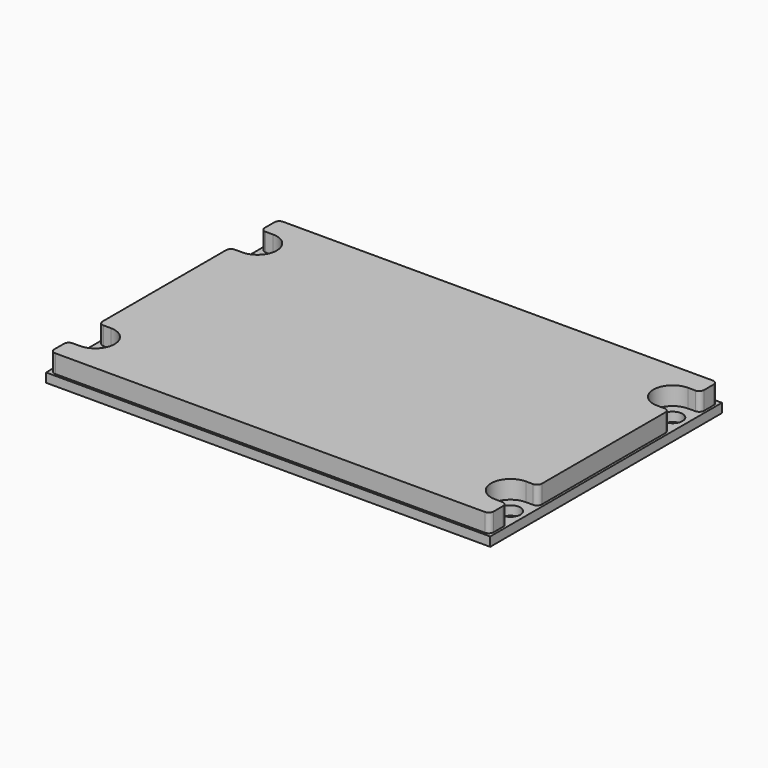
from build123d import *

# Parameters (mm, degrees)
F0_R     = 3.24
F1_DEPTH = 3
F2_DEPTH = 6
F3_R     = 1.588


# Not quite as in the source:
# - a feature names something its author has since deleted; it is built from what else it names


with BuildPart() as f1:
    # F0 (on Top) → F1 (new body)
    with BuildSketch(Plane.XY):
        Polygon((0, 57.15), (-73.025, 57.15), (-73.025, 9.525), (-73.025, -38.1), (73.025, -38.1), (73.025, 57.15), align=None)
        with Locations((-68.262, -23.812)):
            Circle(F0_R, mode=Mode.SUBTRACT)
        with Locations((68.262, -23.812)):
            Circle(F0_R, mode=Mode.SUBTRACT)
        with Locations((-68.262, 42.862)):
            Circle(F0_R, mode=Mode.SUBTRACT)
        with BuildLine():
            Line((-72.225, -17.461), (-72.225, 9.525))
            Line((-72.225, 9.525), (-72.225, 36.511))
            Line((-72.225, 36.511), (-68.262, 36.511))
            ThreePointArc((-68.262, 36.511), (-61.911, 42.862), (-68.262, 49.213))
            Line((-68.262, 49.213), (-72.225, 49.213))
            Line((-72.225, 49.213), (-72.225, 56.35))
            Line((-72.225, 56.35), (72.225, 56.35))
            Line((72.225, 56.35), (72.225, 49.213))
            Line((72.225, 49.213), (68.262, 49.213))
            ThreePointArc((68.262, 49.213), (61.911, 42.862), (68.262, 36.511))
            Line((68.262, 36.511), (72.225, 36.511))
            Line((72.225, 36.511), (72.225, -17.461))
            Line((72.225, -17.461), (68.262, -17.461))
            ThreePointArc((68.262, -17.461), (61.911, -23.812), (68.262, -30.163))
            Line((68.262, -30.163), (72.225, -30.163))
            Line((72.225, -30.163), (72.225, -37.3))
            Line((72.225, -37.3), (-72.225, -37.3))
            Line((-72.225, -37.3), (-72.225, -30.163))
            Line((-72.225, -30.163), (-68.262, -30.163))
            ThreePointArc((-68.262, -30.163), (-61.911, -23.812), (-68.262, -17.461))
            Line((-68.262, -17.461), (-72.225, -17.461))
        make_face(mode=Mode.SUBTRACT)
        with Locations((68.262, 42.862)):
            Circle(F0_R, mode=Mode.SUBTRACT)
        with BuildLine():
            Line((-72.225, 36.511), (-72.225, 9.525))
            Line((-72.225, 9.525), (-72.225, -17.461))
            Line((-72.225, -17.461), (-68.262, -17.461))
            ThreePointArc((-68.262, -17.461), (-61.911, -23.812), (-68.262, -30.163))
            Line((-68.262, -30.163), (-72.225, -30.163))
            Line((-72.225, -30.163), (-72.225, -37.3))
            Line((-72.225, -37.3), (72.225, -37.3))
            Line((72.225, -37.3), (72.225, -30.163))
            Line((72.225, -30.163), (68.262, -30.163))
            ThreePointArc((68.262, -30.163), (61.911, -23.812), (68.262, -17.461))
            Line((68.262, -17.461), (72.225, -17.461))
            Line((72.225, -17.461), (72.225, 36.511))
            Line((72.225, 36.511), (68.262, 36.511))
            ThreePointArc((68.262, 36.511), (61.911, 42.862), (68.262, 49.213))
            Line((68.262, 49.213), (72.225, 49.213))
            Line((72.225, 49.213), (72.225, 56.35))
            Line((72.225, 56.35), (-72.225, 56.35))
            Line((-72.225, 56.35), (-72.225, 49.213))
            Line((-72.225, 49.213), (-68.262, 49.213))
            ThreePointArc((-68.262, 49.213), (-61.911, 42.862), (-68.262, 36.511))
            Line((-68.262, 36.511), (-72.225, 36.511))
        make_face()
    extrude(amount=-F1_DEPTH)


with BuildPart() as f2:
    # F0 (on Top) → F2 (new body)
    with BuildSketch(Plane.XY):
        with BuildLine():
            Line((-72.225, 36.511), (-72.225, 9.525))
            Line((-72.225, 9.525), (-72.225, -17.461))
            Line((-72.225, -17.461), (-68.262, -17.461))
            ThreePointArc((-68.262, -17.461), (-61.911, -23.812), (-68.262, -30.163))
            Line((-68.262, -30.163), (-72.225, -30.163))
            Line((-72.225, -30.163), (-72.225, -37.3))
            Line((-72.225, -37.3), (72.225, -37.3))
            Line((72.225, -37.3), (72.225, -30.163))
            Line((72.225, -30.163), (68.262, -30.163))
            ThreePointArc((68.262, -30.163), (61.911, -23.812), (68.262, -17.461))
            Line((68.262, -17.461), (72.225, -17.461))
            Line((72.225, -17.461), (72.225, 36.511))
            Line((72.225, 36.511), (68.262, 36.511))
            ThreePointArc((68.262, 36.511), (61.911, 42.862), (68.262, 49.213))
            Line((68.262, 49.213), (72.225, 49.213))
            Line((72.225, 49.213), (72.225, 56.35))
            Line((72.225, 56.35), (-72.225, 56.35))
            Line((-72.225, 56.35), (-72.225, 49.213))
            Line((-72.225, 49.213), (-68.262, 49.213))
            ThreePointArc((-68.262, 49.213), (-61.911, 42.862), (-68.262, 36.511))
            Line((-68.262, 36.511), (-72.225, 36.511))
        make_face()
    extrude(amount=F2_DEPTH)

    # F3
    f3_edges = [f2.edges().sort_by_distance(p)[0] for p in [
        (-72.225, 56.35, 3),
        (-72.225, -37.3, 3),
        (72.225, -37.3, 3),
        (72.225, 56.35, 3),
        (-72.225, 36.511, 3),
        (-72.225, -17.461, 3),
        (-72.225, 49.213, 3),
        (72.225, 49.213, 3),
        (72.225, 36.511, 3),
        (72.225, -17.461, 3),
        (72.225, -30.163, 3),
        (-72.225, -30.163, 3),
    ]]
    fillet(f3_edges, radius=F3_R)


solid = Compound([f1.part, f2.part])
